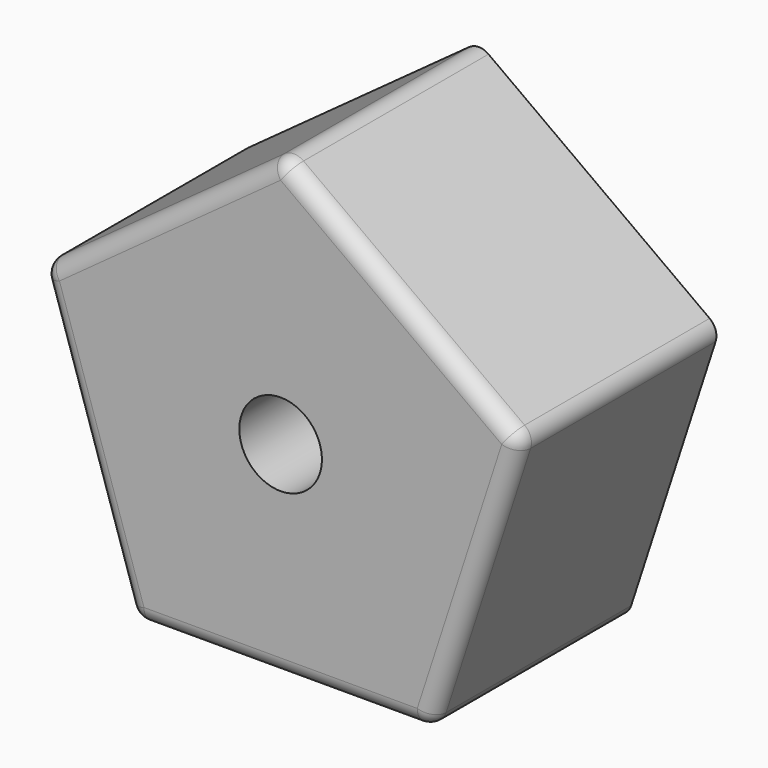
from build123d import *

# Parameters (mm, degrees)
F1_DEPTH     = 76.2
F2_R         = 5.08
F3_T1_DEPTH  = 80.3470901057
F3_T6_DEPTH  = 5.08
F5_T1_DEPTH  = 80.3470901057
F5_T6_DEPTH  = 5.08
F5_T12_DEPTH = 5.08
F6_T1_DEPTH  = 80.3470901057
F6_T6_DEPTH  = 5.08
F6_T12_DEPTH = 5.08
F7_D         = 25.4


# Not quite as in the source:
# - a fillet or chamfer that OpenCascade refuses, or shapes differently, is made with other operations: its cross-section is extruded or revolved along the edge and cut away or added
# - a feature of the source that left no trace in its solid (it failed there, or was rolled back) is left out


with BuildPart() as f1:
    # F0 (on Front) → F1 (new body)
    with BuildSketch(Plane.XZ):
        Polygon((-30.48, -139.1281814039), (-2.2234860344, -52.1635735539), (-76.2, 1.5835099157), (-150.1765139656, -52.1635735539), (-121.92, -139.1281814039), align=None)
    extrude(amount=F1_DEPTH)

    # F2
    f2_edges = [f1.edges().sort_by_distance(p)[0] for p in [
        (-16.351743, -76.2, -95.645877),
        (-39.211743, -76.2, -25.290032),
        (-113.188257, -76.2, -25.290032),
        (-136.048257, -76.2, -95.645877),
        (-76.2, -76.2, -139.128181),
    ]]
    fillet(f2_edges, radius=F2_R)

    # F3: fillet of radius 5.08 on 1 edges, made by hand

    # F3_s2 → F3_t1 (cut)
    with BuildSketch(Plane.XZ.offset(-9.2270901057)):
        with BuildLine():
            ThreePointArc((-149.0359829051, -55.6737672225), (-149.0359829051, -52.5341545596), (-147.190564884, -49.9941545596))
            Line((-147.190564884, -49.9941545596), (-150.1765139656, -52.1635735539))
            Line((-150.1765139656, -52.1635735539), (-149.0359829051, -55.6737672225))
        make_face()
    extrude(amount=F3_T1_DEPTH, mode=Mode.SUBTRACT)


with BuildPart() as f3_tool4:
    # F3_s5 → F3_t6 (new body)
    with BuildSketch(Plane.XZ.offset(71.12)):
        Polygon((-144.2046158024, -54.1039608911), (-149.0359829051, -55.6737672225), (-150.1765139656, -52.1635735539), (-147.190564884, -49.9941545596), align=None)
    extrude(amount=F3_T6_DEPTH)

    # F3_s7 → F3_t8 (revolve, cut)
    with BuildSketch(Plane(origin=(-144.2046158024, -71.12, -54.1039608911), x_dir=(0.9510565163, 0, -0.3090169944), z_dir=(-0.3090169944, 0, -0.9510565163))):
        with BuildLine():
            ThreePointArc((0, -5.08), (5.08, 0), (0, 5.08))
            Line((0, 5.08), (0, -5.08))
        make_face()
    revolve(axis=Axis((-144.2046158024, -71.12, -54.1039608911), (0, -1, 0)), mode=Mode.SUBTRACT)


with BuildPart() as f1_1:
    add(f1.part)

    # F3_t3: cut F3_tool4
    add(f3_tool4.part, mode=Mode.SUBTRACT)

    # F5: fillet of radius 5.08 on 2 edges, made by hand

    # F5_s2 → F5_t1 (cut)
    with BuildSketch(Plane.XZ.offset(-9.2270901057)):
        with BuildLine():
            ThreePointArc((-29.3394689395, -135.6179877354), (-31.1848869606, -138.1579877354), (-34.1708360423, -139.1281814039))
            Line((-34.1708360423, -139.1281814039), (-30.48, -139.1281814039))
            Line((-30.48, -139.1281814039), (-29.3394689395, -135.6179877354))
        make_face()
        with BuildLine():
            ThreePointArc((-3.3640170949, -55.6737672225), (-3.3640170949, -52.5341545596), (-5.209435116, -49.9941545596))
            Line((-5.209435116, -49.9941545596), (-2.2234860344, -52.1635735539))
            Line((-2.2234860344, -52.1635735539), (-3.3640170949, -55.6737672225))
        make_face()
    extrude(amount=F5_T1_DEPTH, mode=Mode.SUBTRACT)


with BuildPart() as f5_tool4:
    # F5_s5 → F5_t6 (new body)
    with BuildSketch(Plane.XZ.offset(71.12)):
        Polygon((-8.1953841976, -54.1039608911), (-3.3640170949, -55.6737672225), (-2.2234860344, -52.1635735539), (-5.209435116, -49.9941545596), align=None)
    extrude(amount=F5_T6_DEPTH)

    # F5_s7 → F5_t8 (revolve, cut)
    with BuildSketch(Plane(origin=(-8.1953841976, -71.12, -54.1039608911), x_dir=(-0.9510565163, 0, -0.3090169944), z_dir=(-0.3090169944, 0, 0.9510565163))):
        with BuildLine():
            ThreePointArc((0, -5.08), (5.08, 0), (0, 5.08))
            Line((0, 5.08), (0, -5.08))
        make_face()
    revolve(axis=Axis((-8.1953841976, -71.12, -54.1039608911), (0, -1, 0)), mode=Mode.SUBTRACT)


with BuildPart() as f1_2:
    add(f1_1.part)

    # F5_t3: cut F5_tool4
    add(f5_tool4.part, mode=Mode.SUBTRACT)


with BuildPart() as f5_tool10:
    # F5_s11 → F5_t12 (new body)
    with BuildSketch(Plane.XZ.offset(71.12)):
        Polygon((-34.1708360423, -134.0481814039), (-29.3394689395, -135.6179877354), (-30.48, -139.1281814039), (-34.1708360423, -139.1281814039), align=None)
    extrude(amount=F5_T12_DEPTH)

    # F5_s13 → F5_t14 (revolve, cut)
    with BuildSketch(Plane(origin=(-34.1708360423, -71.12, -134.0481814039), x_dir=(-0.5877852523, 0, 0.8090169944), z_dir=(0.8090169944, 0, 0.5877852523))):
        with BuildLine():
            ThreePointArc((0, -5.08), (5.08, 0), (0, 5.08))
            Line((0, 5.08), (0, -5.08))
        make_face()
    revolve(axis=Axis((-34.1708360423, -71.12, -134.0481814039), (0, -1, 0)), mode=Mode.SUBTRACT)


with BuildPart() as f1_3:
    add(f1_2.part)

    # F5_t9: cut F5_tool10
    add(f5_tool10.part, mode=Mode.SUBTRACT)

    # F6: fillet of radius 5.08 on 2 edges, made by hand

    # F6_s2 → F6_t1 (cut)
    with BuildSketch(Plane.XZ.offset(-9.2270901057)):
        with BuildLine():
            ThreePointArc((-79.1859490816, -0.5859090786), (-76.2, 0.38428459), (-73.2140509184, -0.5859090786))
            Line((-73.2140509184, -0.5859090786), (-76.2, 1.5835099157))
            Line((-76.2, 1.5835099157), (-79.1859490816, -0.5859090786))
        make_face()
        with BuildLine():
            ThreePointArc((-123.0605310605, -135.6179877354), (-121.2151130394, -138.1579877354), (-118.2291639577, -139.1281814039))
            Line((-118.2291639577, -139.1281814039), (-121.92, -139.1281814039))
            Line((-121.92, -139.1281814039), (-123.0605310605, -135.6179877354))
        make_face()
    extrude(amount=F6_T1_DEPTH, mode=Mode.SUBTRACT)


with BuildPart() as f6_tool4:
    # F6_s5 → F6_t6 (new body)
    with BuildSketch(Plane.XZ.offset(71.12)):
        Polygon((-118.2291639577, -134.0481814039), (-123.0605310605, -135.6179877354), (-121.92, -139.1281814039), (-118.2291639577, -139.1281814039), align=None)
    extrude(amount=F6_T6_DEPTH)

    # F6_s7 → F6_t8 (revolve, cut)
    with BuildSketch(Plane(origin=(-118.2291639577, -71.12, -134.0481814039), x_dir=(0.5877852523, 0, 0.8090169944), z_dir=(0.8090169944, 0, -0.5877852523))):
        with BuildLine():
            ThreePointArc((0, -5.08), (5.08, 0), (0, 5.08))
            Line((0, 5.08), (0, -5.08))
        make_face()
    revolve(axis=Axis((-118.2291639577, -71.12, -134.0481814039), (0, -1, 0)), mode=Mode.SUBTRACT)


with BuildPart() as f1_4:
    add(f1_3.part)

    # F6_t3: cut F6_tool4
    add(f6_tool4.part, mode=Mode.SUBTRACT)


with BuildPart() as f6_tool10:
    # F6_s11 → F6_t12 (new body)
    with BuildSketch(Plane.XZ.offset(71.12)):
        Polygon((-76.2, -4.69571541), (-79.1859490816, -0.5859090786), (-76.2, 1.5835099157), (-73.2140509184, -0.5859090786), align=None)
    extrude(amount=F6_T12_DEPTH)

    # F6_s13 → F6_t14 (revolve, cut)
    with BuildSketch(Plane(origin=(-76.2, -71.12, -4.69571541), x_dir=(0, 0, -1), z_dir=(-1, 0, 0))):
        with BuildLine():
            ThreePointArc((0, -5.08), (5.08, 0), (0, 5.08))
            Line((0, 5.08), (0, -5.08))
        make_face()
    revolve(axis=Axis((-76.2, -71.12, -4.69571541), (0, -1, 0)), mode=Mode.SUBTRACT)


with BuildPart() as f1_5:
    add(f1_4.part)

    # F6_t9: cut F6_tool10
    add(f6_tool10.part, mode=Mode.SUBTRACT)

    # F7 (through all)
    with Locations(Plane(origin=(0, 0, 0), x_dir=(1, 0, 0), z_dir=(0, 1, 0))):
        with Locations((-76.2, 76.2)):
            Hole(F7_D / 2)


solid = f1_5.part
